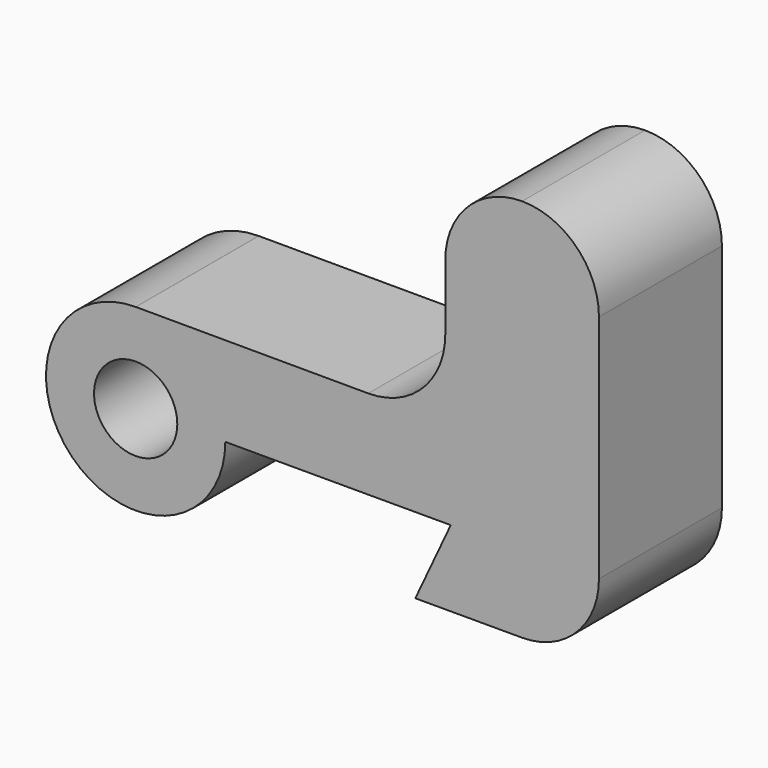
from build123d import *

# Parameters (mm, degrees)
F0_R     = 1.625
F1_DEPTH = 6
F2_R     = 2.99999


# Not quite as in the source:
# - a fillet or chamfer is up to 0.001 mm smaller than in the source, because OpenCascade refuses the exact size


with BuildPart() as f1:
    # F0 (on Front) → F1 (new body)
    with BuildSketch(Plane.XZ):
        with BuildLine():
            Line((12.0862172917, 3.4724390134), (0.0079838936, 3.4999908939))
            ThreePointArc((0.0079838936, 3.4999908939), (0.0039919494, 3.4999977235), (0, 3.5))
            ThreePointArc((0, 3.5), (-2.4748737342, -2.4748737342), (3.5, 0))
            Line((3.5, 0), (12.3, 0))
            Line((12.3, 0), (10.9180201011, -2.9636654571))
            Line((10.9180201011, -2.9636654571), (18.0862172917, -2.9636654571))
            Line((18.0862172917, -2.9636654571), (18.0862172917, 12.0363345429))
            Line((18.0862172917, 12.0363345429), (12.0862172917, 12.0363345429))
            Line((12.0862172917, 12.0363345429), (12.0862172917, 3.4724390134))
        make_face()
        Circle(F0_R, mode=Mode.SUBTRACT)
    extrude(amount=F1_DEPTH)

    # F2 (radius 3 in the source; OpenCascade refuses exactly that, so slightly less here)
    f2_edges = [f1.edges().sort_by_distance(p)[0] for p in [
        (12.086217, -3, 12.036335),
        (12.086217, -3, 3.472439),
        (18.086217, -3, 12.036335),
        (18.086217, -3, -2.963665),
    ]]
    fillet(f2_edges, radius=F2_R)


solid = f1.part
